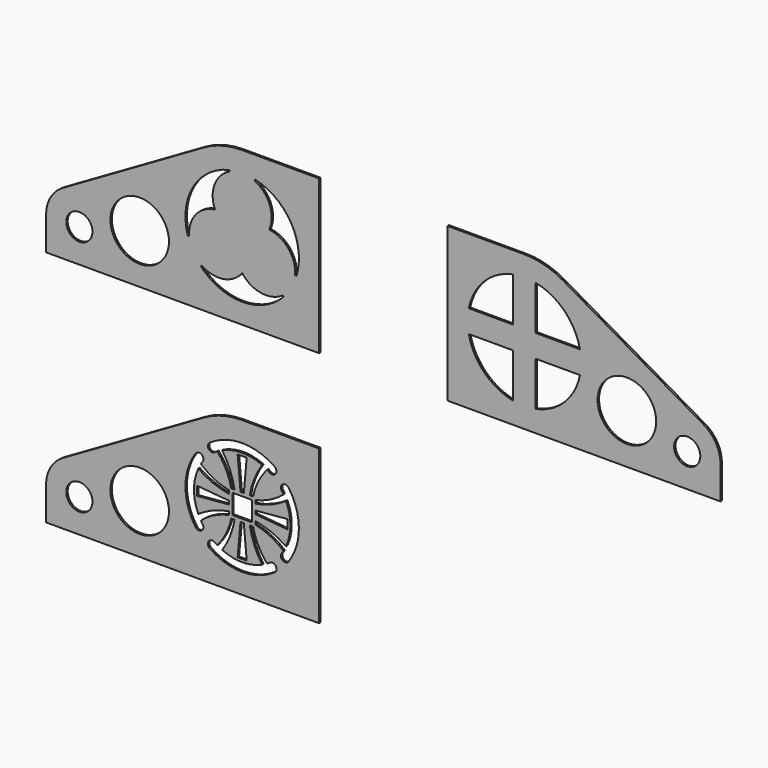
from build123d import *

# Parameters (mm, degrees)
F0_R     = 11.551794
F0_R_2   = 25.800333
F1_DEPTH = 1.6
F2_DEPTH = 1.6
F0_W     = 17.387573
F0_H     = 17.396293
F3_DEPTH = 1.6


# Not quite as in the source:
# - ends of sketch curves that miss each other by under 0.0002 mm in the source are joined


with BuildPart() as f1:
    # F0 (on Front) → F1 (new body)
    with BuildSketch(Plane.XZ):
        with BuildLine():
            Line((-297.186729, 36.993301), (-56.600187, 36.993301))
            Line((-56.600187, 36.993301), (-56.600187, 172.537392))
            Line((-56.600187, 172.537392), (-124.372232, 172.537392))
            ThreePointArc((-124.372232, 172.537392), (-141.9129283344, 170.2281154687), (-158.2582551506, 163.4576592608))
            Line((-158.2582551506, 163.4576592608), (-282.52481, 91.71233))
            ThreePointArc((-282.52481, 91.71233), (-293.2580796825, 80.979060202), (-297.186729, 66.317141))
            Line((-297.186729, 66.317141), (-297.186729, 36.993301))
        make_face()
        with Locations((-267.86289, 66.317141)):
            Circle(F0_R, mode=Mode.SUBTRACT)
        with Locations((-214.686619, 80.56568)):
            Circle(F0_R_2, mode=Mode.SUBTRACT)
        with BuildLine():
            ThreePointArc((-159.9765326971, 71.4023704367), (-141.016905476, 67.0970606221), (-124.3722325089, 77.1448473824))
            ThreePointArc((-124.3722325089, 77.1448473824), (-107.7275592275, 67.0970605743), (-88.7679323029, 71.4023704367))
            Line((-88.7679323029, 71.4023704367), (-87.887164, 70.577047))
            ThreePointArc((-87.887164, 70.577047), (-124.3722323419, 54.765347), (-160.8573001475, 70.5770477988))
            Line((-160.8573001475, 70.5770477988), (-159.9765326971, 71.4023704367))
        make_face(mode=Mode.SUBTRACT)
        with BuildLine():
            ThreePointArc((-172.2227015184, 90.262500146), (-167.6735024781, 129.7653464996), (-135.7376340818, 153.4564923503))
            Line((-135.7376340818, 153.4564923503), (-135.463267, 152.281063))
            ThreePointArc((-135.463267, 152.281063), (-148.6715885036, 138.0141995511), (-148.2922859978, 118.5755964269))
            ThreePointArc((-148.2922859978, 118.5755964269), (-165.3162621194, 109.1847800125), (-171.0675676999, 90.6126060249))
            Line((-171.0675676999, 90.6126060249), (-172.2227015184, 90.262500146))
        make_face(mode=Mode.SUBTRACT)
        with BuildLine():
            ThreePointArc((-77.6768973001, 90.6126060249), (-83.4282028806, 109.1847800125), (-100.4521779276, 118.5755965958))
            ThreePointArc((-100.4521779276, 118.5755965958), (-100.0728755876, 138.0141997906), (-113.2811974601, 152.2810641448))
            Line((-113.2811974601, 152.2810641448), (-113.006831, 153.456492))
            ThreePointArc((-113.006831, 153.456492), (-81.0709616928, 129.7653467957), (-76.5217625658, 90.2624998684))
            Line((-76.5217625658, 90.2624998684), (-77.6768973001, 90.6126060249))
        make_face(mode=Mode.SUBTRACT)
    extrude(amount=F1_DEPTH)


with BuildPart() as f2:
    # F0 (on Front) → F2 (new body)
    with BuildSketch(Plane.XZ):
        with BuildLine():
            ThreePointArc((297.186729, 66.317141), (293.2580796825, 80.979060202), (282.524810096, 91.7123301664))
            Line((282.524810096, 91.7123301664), (158.258255, 163.457659))
            ThreePointArc((158.258255, 163.457659), (141.9129283344, 170.2281154687), (124.372232, 172.537392))
            Line((124.372232, 172.537392), (56.600187, 172.537392))
            Line((56.600187, 172.537392), (56.600187, 36.993301))
            Line((56.600187, 36.993301), (297.186729, 36.993301))
            Line((297.186729, 36.993301), (297.186729, 66.317141))
        make_face()
        with BuildLine():
            ThreePointArc((114.3722320283, 55.7755521386), (89.0168930114, 69.41000787), (75.3824371786, 94.7653468323))
            Line((75.3824371786, 94.7653468323), (114.372232, 94.765347))
            Line((114.372232, 94.765347), (114.3722320283, 55.7755521386))
        make_face(mode=Mode.SUBTRACT)
        with BuildLine():
            ThreePointArc((173.3620268614, 94.7653470283), (159.7275710593, 69.4100079407), (134.3722319717, 55.7755521386))
            Line((134.3722319717, 55.7755521386), (134.372232, 94.765347))
            Line((134.372232, 94.765347), (173.3620268614, 94.7653470283))
        make_face(mode=Mode.SUBTRACT)
        with Locations((214.686619, 80.56568)):
            Circle(F0_R_2, mode=Mode.SUBTRACT)
        with Locations((267.86289, 66.317141)):
            Circle(F0_R, mode=Mode.SUBTRACT)
        with BuildLine():
            Line((114.372232, 114.765347), (75.382438, 114.765347))
            ThreePointArc((75.382438, 114.765347), (89.0168929407, 140.1206860593), (114.3722318323, 153.7551418214))
            Line((114.3722318323, 153.7551418214), (114.372232, 114.765347))
        make_face(mode=Mode.SUBTRACT)
        with BuildLine():
            Line((134.372232, 114.765347), (134.372232, 153.755141))
            ThreePointArc((134.372232, 153.755141), (159.72757113, 140.1206859886), (173.3620268614, 114.7653469717))
            Line((173.3620268614, 114.7653469717), (134.372232, 114.765347))
        make_face(mode=Mode.SUBTRACT)
    extrude(amount=F2_DEPTH)


with BuildPart() as f3:
    # F0 (on Front) → F3 (new body)
    with BuildSketch(Plane.XZ):
        with BuildLine():
            Line((-297.186729, -172.537392), (-56.600187, -172.537392))
            Line((-56.600187, -172.537392), (-56.600187, -36.993301))
            Line((-56.600187, -36.993301), (-124.372232, -36.993301))
            ThreePointArc((-124.372232, -36.993301), (-141.9129280929, -39.3025784666), (-158.2582547176, -46.0730344892))
            Line((-158.2582547176, -46.0730344892), (-282.52481, -117.818363))
            ThreePointArc((-282.52481, -117.818363), (-293.2580796825, -128.551632798), (-297.186729, -143.213552))
            Line((-297.186729, -143.213552), (-297.186729, -172.537392))
        make_face()
        with Locations((-267.86289, -143.213552)):
            Circle(F0_R, mode=Mode.SUBTRACT)
        with Locations((-214.686619, -128.965013)):
            Circle(F0_R_2, mode=Mode.SUBTRACT)
        with BuildLine():
            Line((-136.016088, -111.463298), (-136.016088, -114.409658))
            ThreePointArc((-136.016088, -114.409658), (-149.1748311091, -118.9597856001), (-160.7586581585, -126.6844948177))
            ThreePointArc((-160.7586581585, -126.6844948177), (-160.0034818521, -127.891847864), (-159.2082600619, -129.0732090432))
            ThreePointArc((-159.2082600619, -129.0732090432), (-160.1403536522, -134.3094154984), (-165.3765604984, -133.3773213478))
            ThreePointArc((-165.3765604984, -133.3773213478), (-174.372232, -104.76534659), (-165.3765597693, -76.153372161))
            ThreePointArc((-165.3765597693, -76.153372161), (-160.140353316, -75.2212777363), (-159.2082599709, -80.4574850203))
            ThreePointArc((-159.2082599709, -80.4574850203), (-160.003481619, -81.6388457767), (-160.7586571763, -82.8461984962))
            ThreePointArc((-160.7586571763, -82.8461984962), (-149.1748311091, -90.5709073999), (-136.0160880125, -95.1210350602))
            Line((-136.0160880125, -95.1210350602), (-136.016088, -98.067395))
            ThreePointArc((-136.016088, -98.067395), (-150.1203481061, -94.0894510681), (-163.0175112983, -87.1311919846))
            ThreePointArc((-163.0175112983, -87.1311919846), (-166.850709, -104.7653465451), (-163.0175118922, -122.3994999508))
            ThreePointArc((-163.0175118922, -122.3994999508), (-150.1203481061, -115.4412419319), (-136.016088, -111.463298))
        make_face(mode=Mode.SUBTRACT)
        Polygon((-136.016088, -106.238201), (-164.301496, -108.750682), (-164.301496, -100.780011), (-136.016088, -103.292492), align=None, mode=Mode.SUBTRACT)
        with BuildLine():
            Line((-117.674281, -116.409202), (-114.727921, -116.409202))
            ThreePointArc((-114.727921, -116.409202), (-110.1777933999, -129.5679451091), (-102.4530841823, -141.1517721585))
            ThreePointArc((-102.4530841823, -141.1517721585), (-101.2457306796, -140.3965965559), (-100.0643694875, -139.6013747344))
            ThreePointArc((-100.0643694875, -139.6013747344), (-94.8281635016, -140.5334676522), (-95.7602576522, -145.7696744984))
            ThreePointArc((-95.7602576522, -145.7696744984), (-124.37223241, -154.765347), (-152.9842073083, -145.7696744418))
            ThreePointArc((-152.9842073083, -145.7696744418), (-153.9163012637, -140.533467316), (-148.6800939797, -139.6013739709))
            ThreePointArc((-148.6800939797, -139.6013739709), (-147.4987336797, -140.3965963227), (-146.2913809458, -141.15177191))
            ThreePointArc((-146.2913809458, -141.15177191), (-138.5666716001, -129.5679451091), (-134.0165439398, -116.4092020125))
            Line((-134.0165439398, -116.4092020125), (-131.070184, -116.409202))
            ThreePointArc((-131.070184, -116.409202), (-135.0481279319, -130.5134621061), (-142.0063870154, -143.4106252983))
            ThreePointArc((-142.0063870154, -143.4106252983), (-124.3722324549, -147.243824), (-106.7380786715, -143.4106267199))
            ThreePointArc((-106.7380786715, -143.4106267199), (-113.6963370681, -130.5134621061), (-117.674281, -116.409202))
        make_face(mode=Mode.SUBTRACT)
        Polygon((-122.899378, -116.409202), (-120.386897, -144.69461), (-128.357567, -144.69461), (-125.845087, -116.409202), align=None, mode=Mode.SUBTRACT)
        with Locations((-124.3722325, -104.7653465)):
            Rectangle(F0_W, F0_H, mode=Mode.SUBTRACT)
        Polygon((-112.728377, -103.292492), (-84.442969, -100.780011), (-84.442969, -108.750682), (-112.728377, -106.238201), align=None, mode=Mode.SUBTRACT)
        with BuildLine():
            Line((-112.728377, -98.067395), (-112.728377, -95.121035))
            ThreePointArc((-112.728377, -95.121035), (-99.5696338909, -90.5709073999), (-87.9858068415, -82.8461981823))
            ThreePointArc((-87.9858068415, -82.8461981823), (-88.7409826773, -81.6388453203), (-89.5362042656, -80.4574844875))
            ThreePointArc((-89.5362042656, -80.4574844875), (-88.604111684, -75.2212777363), (-83.3679045016, -76.1533716522))
            ThreePointArc((-83.3679045016, -76.1533716522), (-74.372232, -104.76534659), (-83.3679040889, -133.3773216358))
            ThreePointArc((-83.3679040889, -133.3773216358), (-88.6041113478, -134.3094154984), (-89.5362054984, -129.0732086522))
            ThreePointArc((-89.5362054984, -129.0732086522), (-88.7409824441, -127.8918483204), (-87.985806648, -126.6844952121))
            ThreePointArc((-87.985806648, -126.6844952121), (-99.5696338909, -118.9597856001), (-112.7283769875, -114.4096579398))
            Line((-112.7283769875, -114.4096579398), (-112.728377, -111.463298))
            ThreePointArc((-112.728377, -111.463298), (-98.6241168939, -115.4412419319), (-85.7269537017, -122.3995010154))
            ThreePointArc((-85.7269537017, -122.3995010154), (-81.893755, -104.7653465451), (-85.7269526578, -87.1311928439))
            ThreePointArc((-85.7269526578, -87.1311928439), (-98.6241168939, -94.0894510681), (-112.728377, -98.067395))
        make_face(mode=Mode.SUBTRACT)
        Polygon((-125.845087, -93.121491), (-128.357567, -64.836083), (-120.386897, -64.836083), (-122.899378, -93.121491), align=None, mode=Mode.SUBTRACT)
        with BuildLine():
            Line((-131.070184, -93.121491), (-134.016544, -93.121491))
            ThreePointArc((-134.016544, -93.121491), (-138.5666716001, -79.9627478909), (-146.2913808177, -68.3789208415))
            ThreePointArc((-146.2913808177, -68.3789208415), (-147.4987332233, -69.134097381), (-148.6800940432, -69.9293189381))
            ThreePointArc((-148.6800940432, -69.9293189381), (-153.9163012637, -68.997225684), (-152.9842073478, -63.7610185016))
            ThreePointArc((-152.9842073478, -63.7610185016), (-124.37223241, -54.765347), (-95.7602578335, -63.7610187614))
            ThreePointArc((-95.7602578335, -63.7610187614), (-94.8281635016, -68.9972253478), (-100.0643703478, -69.9293194984))
            ThreePointArc((-100.0643703478, -69.9293194984), (-101.245731136, -69.1340971479), (-102.45308423, -68.3789213817))
            ThreePointArc((-102.45308423, -68.3789213817), (-110.1777933999, -79.9627478909), (-114.7279210602, -93.1214909875))
            Line((-114.7279210602, -93.1214909875), (-117.674281, -93.121491))
            ThreePointArc((-117.674281, -93.121491), (-113.6963370681, -79.0172308939), (-106.7380779846, -66.1200677017))
            ThreePointArc((-106.7380779846, -66.1200677017), (-124.3722324549, -62.28687), (-142.0063857785, -66.1200674855))
            ThreePointArc((-142.0063857785, -66.1200674855), (-135.0481279319, -79.0172308939), (-131.070184, -93.121491))
        make_face(mode=Mode.SUBTRACT)
    extrude(amount=F3_DEPTH)


solid = Compound([f1.part, f2.part, f3.part])
